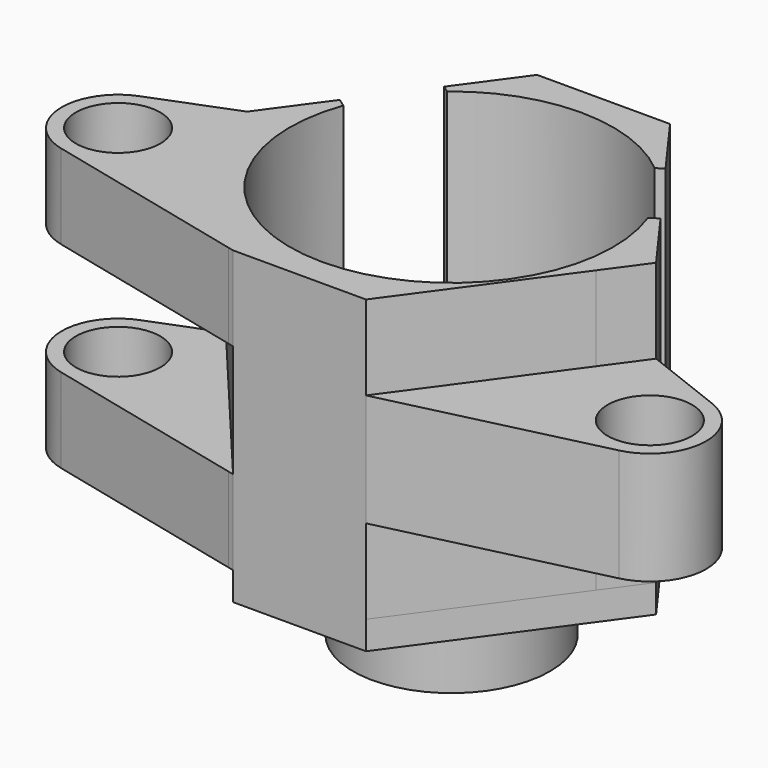
from build123d import *

# Parameters (mm, degrees)
F0_W      = 12.5
F0_H      = 13.5
F0_R      = 5.75
F1_DEPTH  = 5
F3_DEPTH  = 5
F5_DEPTH  = 25
F6_R      = 1.5
F7_DEPTH  = 5
F9_DEPTH  = 1
F10_R     = 1.5
F11_DEPTH = 2
F13_W     = 6.183999799
F13_H     = 4
F14_DEPTH = 25
F17_DEPTH = 10
F20_DEPTH = 25
F21_R     = 3.5
F22_DEPTH = 3


# Not quite as in the source:
# - a feature of the source that left no trace in its solid (it failed there, or was rolled back) is left out
# - a feature names something its author has since deleted; it is built from what else it names


with BuildPart() as f1:
    # F0 (on Top) → F1 (new body, symmetric)
    with BuildSketch(Plane.XY):
        Rectangle(F0_W, F0_H)
        Circle(F0_R, mode=Mode.SUBTRACT)
    extrude(amount=F1_DEPTH, both=True)

    # F2 (on Top) → F3 (join, symmetric)
    with BuildSketch(Plane.XY):
        with BuildLine():
            Line((-4.7552825815, 3.4549150281), (-7.2654252801, 0))
            Line((-7.2654252801, 0), (-4.7552825815, -3.4549150281))
            ThreePointArc((-4.7552825815, -3.4549150281), (-5.8778525229, 0), (-4.7552825815, 3.4549150281))
        make_face()
        with BuildLine():
            Line((4.7552825815, -3.4549150281), (7.2654252801, 0))
            Line((7.2654252801, 0), (4.7552825815, 3.4549150281))
            ThreePointArc((4.7552825815, 3.4549150281), (5.8778525229, 0), (4.7552825815, -3.4549150281))
        make_face()
    extrude(amount=F3_DEPTH, both=True)

    # F4 (on face) → F5 (cut)
    with BuildSketch(Plane.XY.offset(5)):
        Polygon((-8.2530292036, 7.939198947), (-6.25, 1.3976129971), (-1.4972596068, 7.939198947), align=None)
        Polygon((-1.4972596068, -7.939198947), (-6.25, -1.3976129971), (-8.2530292036, -7.939198947), align=None)
        Polygon((8.2530292036, -7.939198947), (6.25, -1.3976129971), (1.4972596068, -7.939198947), align=None)
        Polygon((1.4972596068, 7.939198947), (6.25, 1.3976129971), (8.2530292036, 7.939198947), align=None)
    extrude(amount=-F5_DEPTH, mode=Mode.SUBTRACT)

    # F6 (on Top) → F7 (join, symmetric)
    with BuildSketch(Plane.XY):
        with BuildLine():
            Line((-7.2654252801, 0), (-10.173537518, -1.1373915846))
            ThreePointArc((-10.173537518, -1.1373915846), (-11.4402841733, -3.138029064), (-9.9101168699, -4.9451774907))
            Line((-9.9101168699, -4.9451774907), (-2.5670624157, -6.7007963666))
            Line((-2.5670624157, -6.7007963666), (-2.361263216, -6.75))
            Line((-2.361263216, -6.75), (-7.2654252801, 0))
        make_face()
        with Locations((-9.4450528641, -3)):
            Circle(F6_R, mode=Mode.SUBTRACT)
    extrude(amount=F7_DEPTH, both=True)

    # F8 (on face) → F9 (join)
    with BuildSketch(Plane(origin=(0, 0, -5), x_dir=(1, 0, 0), z_dir=(0, 0, -1))):
        Polygon((2.361263216, -6.75), (7.2654252801, 0), (2.361263216, 6.75), (-2.361263216, 6.75), (-7.2654252801, 0), (-2.361263216, -6.75), align=None)
    extrude(amount=F9_DEPTH)

    # F10 (on Top) → F11 (join, symmetric)
    with BuildSketch(Plane.XY):
        with BuildLine():
            Line((7.2654252801, 0), (2.361263216, -6.75))
            Line((2.361263216, -6.75), (9.9101168699, -4.9451774907))
            ThreePointArc((9.9101168699, -4.9451774907), (11.4402841733, -3.138029064), (10.173537518, -1.1373915846))
            Line((10.173537518, -1.1373915846), (7.2654252801, 0))
        make_face()
        with Locations((9.4450528641, -3)):
            Circle(F10_R, mode=Mode.SUBTRACT)
    extrude(amount=F11_DEPTH, both=True)

    # F13 (on face) → F14 (cut)
    with BuildSketch(Plane(origin=(2.3481090856, -2.7983674386, 0), x_dir=(-0.7660444431, -0.6427876097, 0), z_dir=(-0.6427876097, 0.7660444431, 0))):
        with Locations((9.2396488302, 0)):
            Rectangle(F13_W, F13_H)
    extrude(amount=F14_DEPTH, mode=Mode.SUBTRACT)

    # F16 (on face) → F17 (cut)
    with BuildSketch(Plane.XY.offset(5)):
        Polygon((-6.5190746712, 6.3958671101), (-8.2398039802, 3.9384109772), (-3.2558972089, 0.4486418862), (-1.5351678999, 2.906098019), align=None)
        Polygon((8.2398039802, 3.9384109772), (6.5190746712, 6.3958671101), (1.5351678999, 2.906098019), (3.2558972089, 0.4486418862), align=None)
    extrude(amount=-F17_DEPTH, mode=Mode.SUBTRACT)

    # F19 (on face) → F20 (cut)
    with BuildSketch(Plane(origin=(0, 0, -6), x_dir=(1, 0, 0), z_dir=(0, 0, -1))):
        with BuildLine():
            ThreePointArc((-3.4186985828, 0.75), (-2.4748737342, 2.4748737342), (-0.75, 3.4186985828))
            Line((-0.75, 3.4186985828), (-0.75, 3.9290584114))
            ThreePointArc((-0.75, 3.9290584114), (-2.8284271247, 2.8284271247), (-3.9290584114, 0.75))
            Line((-3.9290584114, 0.75), (-3.4186985828, 0.75))
        make_face()
        with BuildLine():
            Line((0.75, 3.9290584114), (0.75, 3.4186985828))
            ThreePointArc((0.75, 3.4186985828), (2.4748737342, 2.4748737342), (3.4186985828, 0.75))
            Line((3.4186985828, 0.75), (3.9290584114, 0.75))
            ThreePointArc((3.9290584114, 0.75), (2.8284271247, 2.8284271247), (0.75, 3.9290584114))
        make_face()
        with BuildLine():
            Line((-0.75, -3.9290584114), (-0.75, -3.4186985828))
            ThreePointArc((-0.75, -3.4186985828), (-2.4748737342, -2.4748737342), (-3.4186985828, -0.75))
            Line((-3.4186985828, -0.75), (-3.9290584114, -0.75))
            ThreePointArc((-3.9290584114, -0.75), (-2.8284271247, -2.8284271247), (-0.75, -3.9290584114))
        make_face()
        with BuildLine():
            ThreePointArc((3.4186985828, -0.75), (2.4748737342, -2.4748737342), (0.75, -3.4186985828))
            Line((0.75, -3.4186985828), (0.75, -3.9290584114))
            ThreePointArc((0.75, -3.9290584114), (2.8284271247, -2.8284271247), (3.9290584114, -0.75))
            Line((3.9290584114, -0.75), (3.4186985828, -0.75))
        make_face()
    extrude(amount=-F20_DEPTH, mode=Mode.SUBTRACT)

    # F21 (on face) → F22 (join)
    with BuildSketch(Plane(origin=(0, 0, -6), x_dir=(1, 0, 0), z_dir=(0, 0, -1))):
        Circle(F21_R)
    extrude(amount=F22_DEPTH)


solid = f1.part
